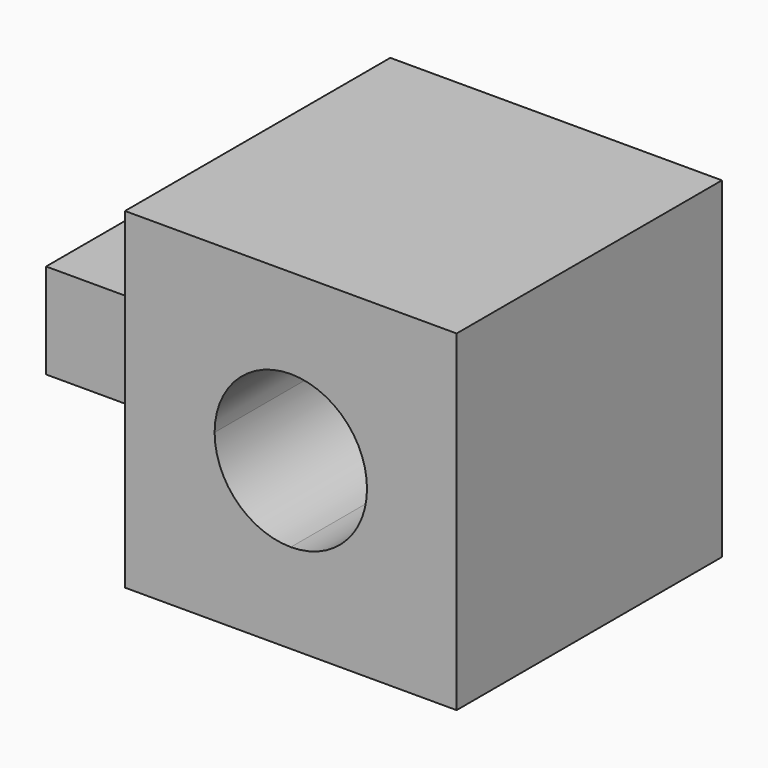
from build123d import *

# Parameters (mm, degrees)
F1_DEPTH = 50.8
F3_DEPTH = 25.4


# Not quite as in the source:
# - a feature names something its author has since deleted; it is built from what else it names


with BuildPart() as f1:
    # F0 (on Front) → F1 (new body)
    with BuildSketch(Plane.XZ):
        with BuildLine():
            Line((-37.0038875103, 50.8), (-62.4038875103, 50.8))
            Line((-62.4038875103, 50.8), (-62.4038875103, 25.4))
            Line((-62.4038875103, 25.4), (-48.6759059699, 25.4))
            ThreePointArc((-48.6759059699, 25.4), (-45.2572509132, 33.6533634029), (-37.0038875103, 37.0720184596))
            Line((-37.0038875103, 37.0720184596), (-37.0038875103, 50.8))
        make_face()
        with BuildLine():
            Line((-48.6759059699, 25.4), (-62.4038875103, 25.4))
            Line((-62.4038875103, 25.4), (-62.4038875103, 0))
            Line((-62.4038875103, 0), (-37.0038875103, 0))
            Line((-37.0038875103, 0), (-37.0038875103, 13.7279815404))
            ThreePointArc((-37.0038875103, 13.7279815404), (-45.2572509132, 17.1466365971), (-48.6759059699, 25.4))
        make_face()
        with BuildLine():
            Line((-11.6038875103, 50.8), (-37.0038875103, 50.8))
            Line((-37.0038875103, 50.8), (-37.0038875103, 37.0720184596))
            ThreePointArc((-37.0038875103, 37.0720184596), (-28.7505241074, 33.6533634029), (-25.3318690507, 25.4))
            Line((-25.3318690507, 25.4), (-11.6038875103, 25.4))
            Line((-11.6038875103, 25.4), (-11.6038875103, 50.8))
        make_face()
        with BuildLine():
            Line((-37.0038875103, 13.7279815404), (-37.0038875103, 0))
            Line((-37.0038875103, 0), (-11.6038875103, 0))
            Line((-11.6038875103, 0), (-11.6038875103, 25.4))
            Line((-11.6038875103, 25.4), (-25.3318690507, 25.4))
            ThreePointArc((-25.3318690507, 25.4), (-28.7505241074, 17.1466365971), (-37.0038875103, 13.7279815404))
        make_face()
    extrude(amount=F1_DEPTH)

    # F2 (on face) → F3 (join)
    with BuildSketch(Plane(origin=(-62.4038875103, 0, 0), x_dir=(0, -1, 0), z_dir=(-1, 0, 0))):
        Polygon((16.7379435152, 28.2901115716), (17.1399507672, 13.7242572382), (34.1606251895, 13.7242572382), (34.1606251895, 28.2901115716), align=None)
    extrude(amount=F3_DEPTH)


solid = f1.part
